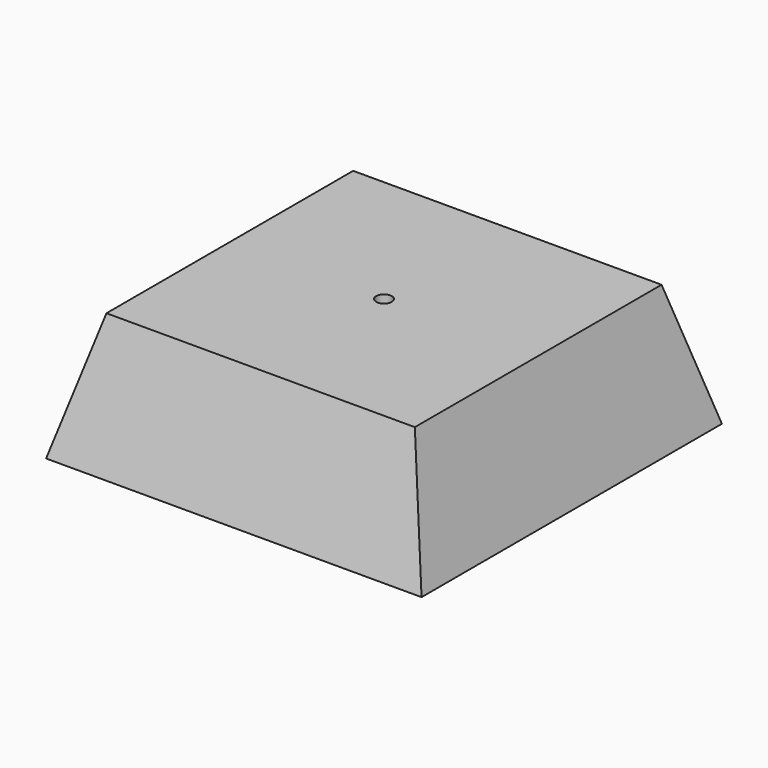
from build123d import *

# Parameters (mm, degrees)
F0_W     = 152.4
F0_H     = 152.4
F0_R     = 3.175
F1_DEPTH = 50.8
F2_SIZE2 = 13.611809
F2_SIZE  = 50.79999


# Not quite as in the source:
# - a fillet or chamfer is up to 0.001 mm smaller than in the source, because OpenCascade refuses the exact size
# - a feature names something its author has since deleted; it is built from what else it names


with BuildPart() as f1:
    # F0 (on Top) → F1 (new body)
    with BuildSketch(Plane.XY):
        with Locations((76.2, 76.2)):
            Rectangle(F0_W, F0_H)
        with Locations((76.2, 76.2)):
            Circle(F0_R, mode=Mode.SUBTRACT)
    extrude(amount=F1_DEPTH)

    # F2 (size 50.8 and 13.6118189755 in the source; OpenCascade refuses exactly that, so slightly less here)
    f2_edges = [f1.edges().sort_by_distance(p)[0] for p in [
        (0, 76.2, 50.8),
        (76.2, 152.4, 50.8),
        (152.4, 76.2, 50.8),
        (76.2, 0, 50.8),
    ]]
    chamfer(f2_edges, length=F2_SIZE, length2=F2_SIZE2)


solid = f1.part
